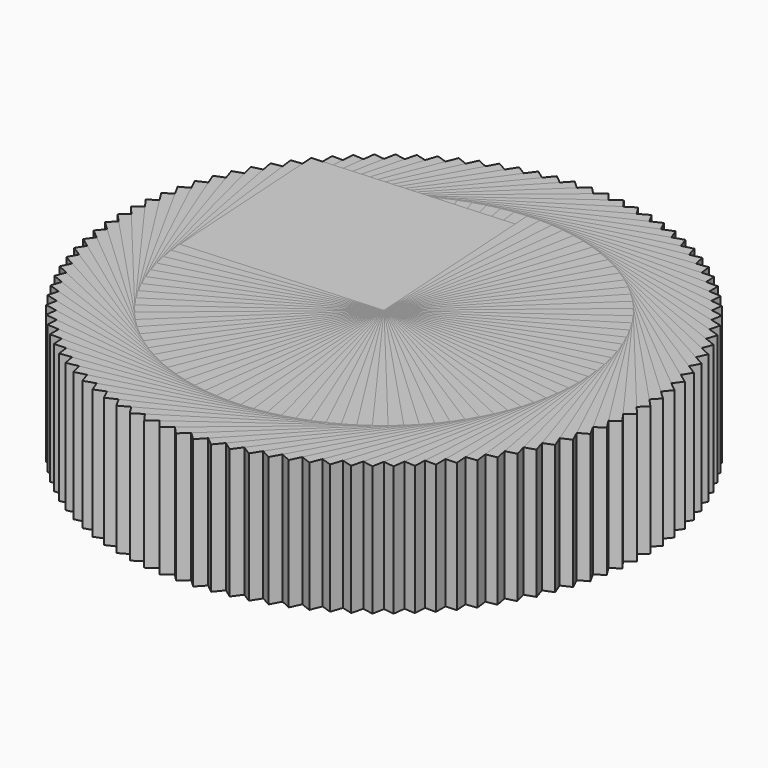
from build123d import *

# Parameters (mm, degrees)
F0_W     = 60
F0_H     = 55
F1_DEPTH = 40
F2_COUNT = 100


with BuildPart() as f1:
    # F0 (on Top) → F1 (new body)
    with BuildSketch(Plane.XY):
        with Locations((-30, 27.5)):
            Rectangle(F0_W, F0_H)
    extrude(amount=F1_DEPTH)


with BuildPart() as f2_1:
    # F2: instance of F1
    add(f1.part.rotate(Axis((0, 0, 20), (0, 0, -1)), 1 * 360 / F2_COUNT))


with BuildPart() as f2_2:
    # F2: instance of F1
    add(f1.part.rotate(Axis((0, 0, 20), (0, 0, -1)), 2 * 360 / F2_COUNT))


with BuildPart() as f2_3:
    # F2: instance of F1
    add(f1.part.rotate(Axis((0, 0, 20), (0, 0, -1)), 3 * 360 / F2_COUNT))


with BuildPart() as f2_4:
    # F2: instance of F1
    add(f1.part.rotate(Axis((0, 0, 20), (0, 0, -1)), 4 * 360 / F2_COUNT))


with BuildPart() as f2_5:
    # F2: instance of F1
    add(f1.part.rotate(Axis((0, 0, 20), (0, 0, -1)), 5 * 360 / F2_COUNT))


with BuildPart() as f2_6:
    # F2: instance of F1
    add(f1.part.rotate(Axis((0, 0, 20), (0, 0, -1)), 6 * 360 / F2_COUNT))


with BuildPart() as f2_7:
    # F2: instance of F1
    add(f1.part.rotate(Axis((0, 0, 20), (0, 0, -1)), 7 * 360 / F2_COUNT))


with BuildPart() as f2_8:
    # F2: instance of F1
    add(f1.part.rotate(Axis((0, 0, 20), (0, 0, -1)), 8 * 360 / F2_COUNT))


with BuildPart() as f2_9:
    # F2: instance of F1
    add(f1.part.rotate(Axis((0, 0, 20), (0, 0, -1)), 9 * 360 / F2_COUNT))


with BuildPart() as f2_10:
    # F2: instance of F1
    add(f1.part.rotate(Axis((0, 0, 20), (0, 0, -1)), 10 * 360 / F2_COUNT))


with BuildPart() as f2_11:
    # F2: instance of F1
    add(f1.part.rotate(Axis((0, 0, 20), (0, 0, -1)), 11 * 360 / F2_COUNT))


with BuildPart() as f2_12:
    # F2: instance of F1
    add(f1.part.rotate(Axis((0, 0, 20), (0, 0, -1)), 12 * 360 / F2_COUNT))


with BuildPart() as f2_13:
    # F2: instance of F1
    add(f1.part.rotate(Axis((0, 0, 20), (0, 0, -1)), 13 * 360 / F2_COUNT))


with BuildPart() as f2_14:
    # F2: instance of F1
    add(f1.part.rotate(Axis((0, 0, 20), (0, 0, -1)), 14 * 360 / F2_COUNT))


with BuildPart() as f2_15:
    # F2: instance of F1
    add(f1.part.rotate(Axis((0, 0, 20), (0, 0, -1)), 15 * 360 / F2_COUNT))


with BuildPart() as f2_16:
    # F2: instance of F1
    add(f1.part.rotate(Axis((0, 0, 20), (0, 0, -1)), 16 * 360 / F2_COUNT))


with BuildPart() as f2_17:
    # F2: instance of F1
    add(f1.part.rotate(Axis((0, 0, 20), (0, 0, -1)), 17 * 360 / F2_COUNT))


with BuildPart() as f2_18:
    # F2: instance of F1
    add(f1.part.rotate(Axis((0, 0, 20), (0, 0, -1)), 18 * 360 / F2_COUNT))


with BuildPart() as f2_19:
    # F2: instance of F1
    add(f1.part.rotate(Axis((0, 0, 20), (0, 0, -1)), 19 * 360 / F2_COUNT))


with BuildPart() as f2_20:
    # F2: instance of F1
    add(f1.part.rotate(Axis((0, 0, 20), (0, 0, -1)), 20 * 360 / F2_COUNT))


with BuildPart() as f2_21:
    # F2: instance of F1
    add(f1.part.rotate(Axis((0, 0, 20), (0, 0, -1)), 21 * 360 / F2_COUNT))


with BuildPart() as f2_22:
    # F2: instance of F1
    add(f1.part.rotate(Axis((0, 0, 20), (0, 0, -1)), 22 * 360 / F2_COUNT))


with BuildPart() as f2_23:
    # F2: instance of F1
    add(f1.part.rotate(Axis((0, 0, 20), (0, 0, -1)), 23 * 360 / F2_COUNT))


with BuildPart() as f2_24:
    # F2: instance of F1
    add(f1.part.rotate(Axis((0, 0, 20), (0, 0, -1)), 24 * 360 / F2_COUNT))


with BuildPart() as f2_25:
    # F2: instance of F1
    add(f1.part.rotate(Axis((0, 0, 20), (0, 0, -1)), 25 * 360 / F2_COUNT))


with BuildPart() as f2_26:
    # F2: instance of F1
    add(f1.part.rotate(Axis((0, 0, 20), (0, 0, -1)), 26 * 360 / F2_COUNT))


with BuildPart() as f2_27:
    # F2: instance of F1
    add(f1.part.rotate(Axis((0, 0, 20), (0, 0, -1)), 27 * 360 / F2_COUNT))


with BuildPart() as f2_28:
    # F2: instance of F1
    add(f1.part.rotate(Axis((0, 0, 20), (0, 0, -1)), 28 * 360 / F2_COUNT))


with BuildPart() as f2_29:
    # F2: instance of F1
    add(f1.part.rotate(Axis((0, 0, 20), (0, 0, -1)), 29 * 360 / F2_COUNT))


with BuildPart() as f2_30:
    # F2: instance of F1
    add(f1.part.rotate(Axis((0, 0, 20), (0, 0, -1)), 30 * 360 / F2_COUNT))


with BuildPart() as f2_31:
    # F2: instance of F1
    add(f1.part.rotate(Axis((0, 0, 20), (0, 0, -1)), 31 * 360 / F2_COUNT))


with BuildPart() as f2_32:
    # F2: instance of F1
    add(f1.part.rotate(Axis((0, 0, 20), (0, 0, -1)), 32 * 360 / F2_COUNT))


with BuildPart() as f2_33:
    # F2: instance of F1
    add(f1.part.rotate(Axis((0, 0, 20), (0, 0, -1)), 33 * 360 / F2_COUNT))


with BuildPart() as f2_34:
    # F2: instance of F1
    add(f1.part.rotate(Axis((0, 0, 20), (0, 0, -1)), 34 * 360 / F2_COUNT))


with BuildPart() as f2_35:
    # F2: instance of F1
    add(f1.part.rotate(Axis((0, 0, 20), (0, 0, -1)), 35 * 360 / F2_COUNT))


with BuildPart() as f2_36:
    # F2: instance of F1
    add(f1.part.rotate(Axis((0, 0, 20), (0, 0, -1)), 36 * 360 / F2_COUNT))


with BuildPart() as f2_37:
    # F2: instance of F1
    add(f1.part.rotate(Axis((0, 0, 20), (0, 0, -1)), 37 * 360 / F2_COUNT))


with BuildPart() as f2_38:
    # F2: instance of F1
    add(f1.part.rotate(Axis((0, 0, 20), (0, 0, -1)), 38 * 360 / F2_COUNT))


with BuildPart() as f2_39:
    # F2: instance of F1
    add(f1.part.rotate(Axis((0, 0, 20), (0, 0, -1)), 39 * 360 / F2_COUNT))


with BuildPart() as f2_40:
    # F2: instance of F1
    add(f1.part.rotate(Axis((0, 0, 20), (0, 0, -1)), 40 * 360 / F2_COUNT))


with BuildPart() as f2_41:
    # F2: instance of F1
    add(f1.part.rotate(Axis((0, 0, 20), (0, 0, -1)), 41 * 360 / F2_COUNT))


with BuildPart() as f2_42:
    # F2: instance of F1
    add(f1.part.rotate(Axis((0, 0, 20), (0, 0, -1)), 42 * 360 / F2_COUNT))


with BuildPart() as f2_43:
    # F2: instance of F1
    add(f1.part.rotate(Axis((0, 0, 20), (0, 0, -1)), 43 * 360 / F2_COUNT))


with BuildPart() as f2_44:
    # F2: instance of F1
    add(f1.part.rotate(Axis((0, 0, 20), (0, 0, -1)), 44 * 360 / F2_COUNT))


with BuildPart() as f2_45:
    # F2: instance of F1
    add(f1.part.rotate(Axis((0, 0, 20), (0, 0, -1)), 45 * 360 / F2_COUNT))


with BuildPart() as f2_46:
    # F2: instance of F1
    add(f1.part.rotate(Axis((0, 0, 20), (0, 0, -1)), 46 * 360 / F2_COUNT))


with BuildPart() as f2_47:
    # F2: instance of F1
    add(f1.part.rotate(Axis((0, 0, 20), (0, 0, -1)), 47 * 360 / F2_COUNT))


with BuildPart() as f2_48:
    # F2: instance of F1
    add(f1.part.rotate(Axis((0, 0, 20), (0, 0, -1)), 48 * 360 / F2_COUNT))


with BuildPart() as f2_49:
    # F2: instance of F1
    add(f1.part.rotate(Axis((0, 0, 20), (0, 0, -1)), 49 * 360 / F2_COUNT))


with BuildPart() as f2_50:
    # F2: instance of F1
    add(f1.part.rotate(Axis((0, 0, 20), (0, 0, -1)), 50 * 360 / F2_COUNT))


with BuildPart() as f2_51:
    # F2: instance of F1
    add(f1.part.rotate(Axis((0, 0, 20), (0, 0, -1)), 51 * 360 / F2_COUNT))


with BuildPart() as f2_52:
    # F2: instance of F1
    add(f1.part.rotate(Axis((0, 0, 20), (0, 0, -1)), 52 * 360 / F2_COUNT))


with BuildPart() as f2_53:
    # F2: instance of F1
    add(f1.part.rotate(Axis((0, 0, 20), (0, 0, -1)), 53 * 360 / F2_COUNT))


with BuildPart() as f2_54:
    # F2: instance of F1
    add(f1.part.rotate(Axis((0, 0, 20), (0, 0, -1)), 54 * 360 / F2_COUNT))


with BuildPart() as f2_55:
    # F2: instance of F1
    add(f1.part.rotate(Axis((0, 0, 20), (0, 0, -1)), 55 * 360 / F2_COUNT))


with BuildPart() as f2_56:
    # F2: instance of F1
    add(f1.part.rotate(Axis((0, 0, 20), (0, 0, -1)), 56 * 360 / F2_COUNT))


with BuildPart() as f2_57:
    # F2: instance of F1
    add(f1.part.rotate(Axis((0, 0, 20), (0, 0, -1)), 57 * 360 / F2_COUNT))


with BuildPart() as f2_58:
    # F2: instance of F1
    add(f1.part.rotate(Axis((0, 0, 20), (0, 0, -1)), 58 * 360 / F2_COUNT))


with BuildPart() as f2_59:
    # F2: instance of F1
    add(f1.part.rotate(Axis((0, 0, 20), (0, 0, -1)), 59 * 360 / F2_COUNT))


with BuildPart() as f2_60:
    # F2: instance of F1
    add(f1.part.rotate(Axis((0, 0, 20), (0, 0, -1)), 60 * 360 / F2_COUNT))


with BuildPart() as f2_61:
    # F2: instance of F1
    add(f1.part.rotate(Axis((0, 0, 20), (0, 0, -1)), 61 * 360 / F2_COUNT))


with BuildPart() as f2_62:
    # F2: instance of F1
    add(f1.part.rotate(Axis((0, 0, 20), (0, 0, -1)), 62 * 360 / F2_COUNT))


with BuildPart() as f2_63:
    # F2: instance of F1
    add(f1.part.rotate(Axis((0, 0, 20), (0, 0, -1)), 63 * 360 / F2_COUNT))


with BuildPart() as f2_64:
    # F2: instance of F1
    add(f1.part.rotate(Axis((0, 0, 20), (0, 0, -1)), 64 * 360 / F2_COUNT))


with BuildPart() as f2_65:
    # F2: instance of F1
    add(f1.part.rotate(Axis((0, 0, 20), (0, 0, -1)), 65 * 360 / F2_COUNT))


with BuildPart() as f2_66:
    # F2: instance of F1
    add(f1.part.rotate(Axis((0, 0, 20), (0, 0, -1)), 66 * 360 / F2_COUNT))


with BuildPart() as f2_67:
    # F2: instance of F1
    add(f1.part.rotate(Axis((0, 0, 20), (0, 0, -1)), 67 * 360 / F2_COUNT))


with BuildPart() as f2_68:
    # F2: instance of F1
    add(f1.part.rotate(Axis((0, 0, 20), (0, 0, -1)), 68 * 360 / F2_COUNT))


with BuildPart() as f2_69:
    # F2: instance of F1
    add(f1.part.rotate(Axis((0, 0, 20), (0, 0, -1)), 69 * 360 / F2_COUNT))


with BuildPart() as f2_70:
    # F2: instance of F1
    add(f1.part.rotate(Axis((0, 0, 20), (0, 0, -1)), 70 * 360 / F2_COUNT))


with BuildPart() as f2_71:
    # F2: instance of F1
    add(f1.part.rotate(Axis((0, 0, 20), (0, 0, -1)), 71 * 360 / F2_COUNT))


with BuildPart() as f2_72:
    # F2: instance of F1
    add(f1.part.rotate(Axis((0, 0, 20), (0, 0, -1)), 72 * 360 / F2_COUNT))


with BuildPart() as f2_73:
    # F2: instance of F1
    add(f1.part.rotate(Axis((0, 0, 20), (0, 0, -1)), 73 * 360 / F2_COUNT))


with BuildPart() as f2_74:
    # F2: instance of F1
    add(f1.part.rotate(Axis((0, 0, 20), (0, 0, -1)), 74 * 360 / F2_COUNT))


with BuildPart() as f2_75:
    # F2: instance of F1
    add(f1.part.rotate(Axis((0, 0, 20), (0, 0, -1)), 75 * 360 / F2_COUNT))


with BuildPart() as f2_76:
    # F2: instance of F1
    add(f1.part.rotate(Axis((0, 0, 20), (0, 0, -1)), 76 * 360 / F2_COUNT))


with BuildPart() as f2_77:
    # F2: instance of F1
    add(f1.part.rotate(Axis((0, 0, 20), (0, 0, -1)), 77 * 360 / F2_COUNT))


with BuildPart() as f2_78:
    # F2: instance of F1
    add(f1.part.rotate(Axis((0, 0, 20), (0, 0, -1)), 78 * 360 / F2_COUNT))


with BuildPart() as f2_79:
    # F2: instance of F1
    add(f1.part.rotate(Axis((0, 0, 20), (0, 0, -1)), 79 * 360 / F2_COUNT))


with BuildPart() as f2_80:
    # F2: instance of F1
    add(f1.part.rotate(Axis((0, 0, 20), (0, 0, -1)), 80 * 360 / F2_COUNT))


with BuildPart() as f2_81:
    # F2: instance of F1
    add(f1.part.rotate(Axis((0, 0, 20), (0, 0, -1)), 81 * 360 / F2_COUNT))


with BuildPart() as f2_82:
    # F2: instance of F1
    add(f1.part.rotate(Axis((0, 0, 20), (0, 0, -1)), 82 * 360 / F2_COUNT))


with BuildPart() as f2_83:
    # F2: instance of F1
    add(f1.part.rotate(Axis((0, 0, 20), (0, 0, -1)), 83 * 360 / F2_COUNT))


with BuildPart() as f2_84:
    # F2: instance of F1
    add(f1.part.rotate(Axis((0, 0, 20), (0, 0, -1)), 84 * 360 / F2_COUNT))


with BuildPart() as f2_85:
    # F2: instance of F1
    add(f1.part.rotate(Axis((0, 0, 20), (0, 0, -1)), 85 * 360 / F2_COUNT))


with BuildPart() as f2_86:
    # F2: instance of F1
    add(f1.part.rotate(Axis((0, 0, 20), (0, 0, -1)), 86 * 360 / F2_COUNT))


with BuildPart() as f2_87:
    # F2: instance of F1
    add(f1.part.rotate(Axis((0, 0, 20), (0, 0, -1)), 87 * 360 / F2_COUNT))


with BuildPart() as f2_88:
    # F2: instance of F1
    add(f1.part.rotate(Axis((0, 0, 20), (0, 0, -1)), 88 * 360 / F2_COUNT))


with BuildPart() as f2_89:
    # F2: instance of F1
    add(f1.part.rotate(Axis((0, 0, 20), (0, 0, -1)), 89 * 360 / F2_COUNT))


with BuildPart() as f2_90:
    # F2: instance of F1
    add(f1.part.rotate(Axis((0, 0, 20), (0, 0, -1)), 90 * 360 / F2_COUNT))


with BuildPart() as f2_91:
    # F2: instance of F1
    add(f1.part.rotate(Axis((0, 0, 20), (0, 0, -1)), 91 * 360 / F2_COUNT))


with BuildPart() as f2_92:
    # F2: instance of F1
    add(f1.part.rotate(Axis((0, 0, 20), (0, 0, -1)), 92 * 360 / F2_COUNT))


with BuildPart() as f2_93:
    # F2: instance of F1
    add(f1.part.rotate(Axis((0, 0, 20), (0, 0, -1)), 93 * 360 / F2_COUNT))


with BuildPart() as f2_94:
    # F2: instance of F1
    add(f1.part.rotate(Axis((0, 0, 20), (0, 0, -1)), 94 * 360 / F2_COUNT))


with BuildPart() as f2_95:
    # F2: instance of F1
    add(f1.part.rotate(Axis((0, 0, 20), (0, 0, -1)), 95 * 360 / F2_COUNT))


with BuildPart() as f2_96:
    # F2: instance of F1
    add(f1.part.rotate(Axis((0, 0, 20), (0, 0, -1)), 96 * 360 / F2_COUNT))


with BuildPart() as f2_97:
    # F2: instance of F1
    add(f1.part.rotate(Axis((0, 0, 20), (0, 0, -1)), 97 * 360 / F2_COUNT))


with BuildPart() as f2_98:
    # F2: instance of F1
    add(f1.part.rotate(Axis((0, 0, 20), (0, 0, -1)), 98 * 360 / F2_COUNT))


with BuildPart() as f2_99:
    # F2: instance of F1
    add(f1.part.rotate(Axis((0, 0, 20), (0, 0, -1)), 99 * 360 / F2_COUNT))


solid = Compound([f1.part, f2_1.part, f2_2.part, f2_3.part, f2_4.part, f2_5.part, f2_6.part, f2_7.part, f2_8.part, f2_9.part, f2_10.part, f2_11.part, f2_12.part, f2_13.part, f2_14.part, f2_15.part, f2_16.part, f2_17.part, f2_18.part, f2_19.part, f2_20.part, f2_21.part, f2_22.part, f2_23.part, f2_24.part, f2_25.part, f2_26.part, f2_27.part, f2_28.part, f2_29.part, f2_30.part, f2_31.part, f2_32.part, f2_33.part, f2_34.part, f2_35.part, f2_36.part, f2_37.part, f2_38.part, f2_39.part, f2_40.part, f2_41.part, f2_42.part, f2_43.part, f2_44.part, f2_45.part, f2_46.part, f2_47.part, f2_48.part, f2_49.part, f2_50.part, f2_51.part, f2_52.part, f2_53.part, f2_54.part, f2_55.part, f2_56.part, f2_57.part, f2_58.part, f2_59.part, f2_60.part, f2_61.part, f2_62.part, f2_63.part, f2_64.part, f2_65.part, f2_66.part, f2_67.part, f2_68.part, f2_69.part, f2_70.part, f2_71.part, f2_72.part, f2_73.part, f2_74.part, f2_75.part, f2_76.part, f2_77.part, f2_78.part, f2_79.part, f2_80.part, f2_81.part, f2_82.part, f2_83.part, f2_84.part, f2_85.part, f2_86.part, f2_87.part, f2_88.part, f2_89.part, f2_90.part, f2_91.part, f2_92.part, f2_93.part, f2_94.part, f2_95.part, f2_96.part, f2_97.part, f2_98.part, f2_99.part])
